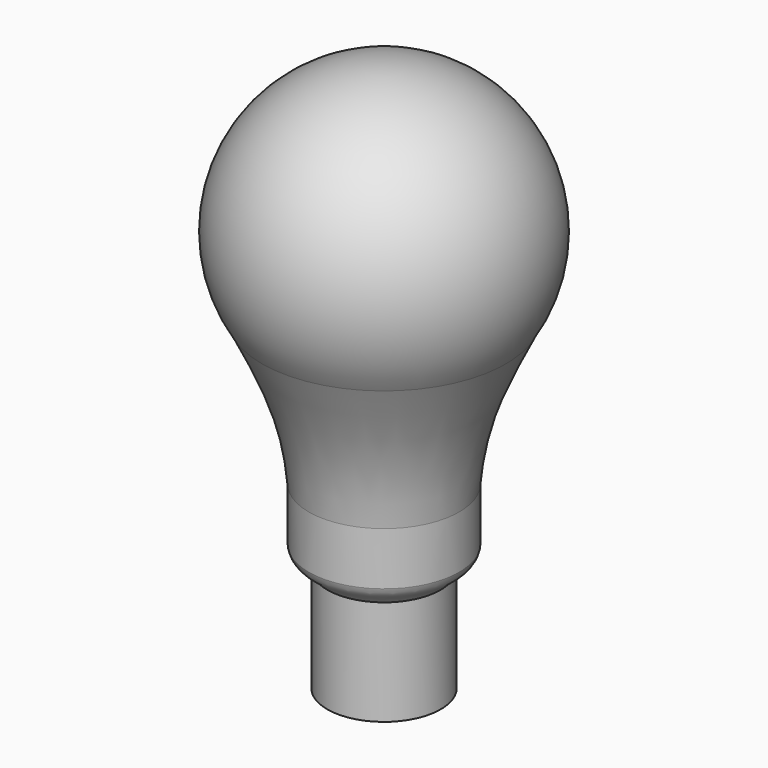
from build123d import *


# Not quite as in the source:
# - a feature names something its author has since deleted; it is built from what else it names


with BuildPart() as f1:
    # F0 (on Front) → F1 (revolve)
    with BuildSketch(Plane.XZ):
        with BuildLine():
            Line((0, -3.5306), (0, 0))
            Line((0, 0), (0, 29.7434))
            Line((0, 29.7434), (0, 63.0174))
            ThreePointArc((0, 63.0174), (-29.1585229497, 45.772736087), (-28.0935123016, 11.9132670067))
            ThreePointArc((-28.0935123016, 11.9132670067), (-16.029336087, 0.5848770503), (0, -3.5306))
        make_face()
        with BuildLine():
            Line((0, -38.7858), (0, -3.5306))
            ThreePointArc((0, -3.5306), (-16.029336087, 0.5848770503), (-28.0935123016, 11.9132670067))
            add(Edge.make_bspline(
                [(-17.3482, -21.60576857), (-18.3633640409, -8.3696646616), (-22.1754945815, 0), (-28.0935123016, 11.9132670067)],
                knots=[0, 0, 0, 0, 35.1992540043, 35.1992540043, 35.1992540043, 35.1992540043], degree=3))
            Line((-17.3482, -21.60576857), (-17.3482, -33.7980993547))
            add(Edge.make_bspline(
                [(-17.3482, -33.7980993547), (-16.8019030243, -36.5484394133), (-14.2998911163, -36.8996322387), (-13.081, -38.7858)],
                knots=[0, 0, 0, 0, 6.5640043851, 6.5640043851, 6.5640043851, 6.5640043851], degree=3))
            Line((-13.081, -38.7858), (-13.081, -63.0174))
            Line((-13.081, -63.0174), (0, -63.0174))
            Line((0, -63.0174), (0, -38.7858))
        make_face()
    revolve(axis=Axis((0, 0, 31.5087), (0, 0, 1)))


solid = f1.part
